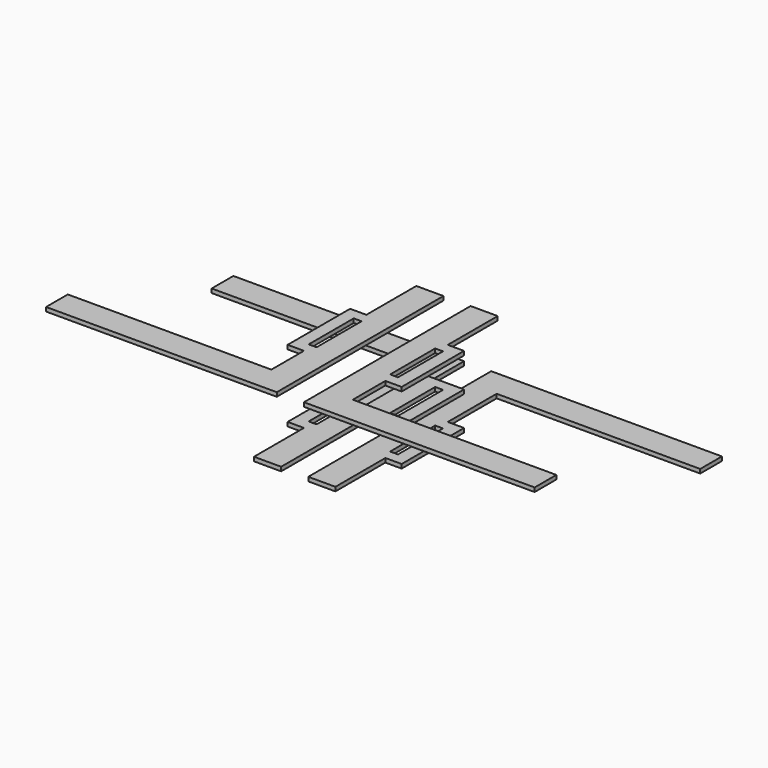
from build123d import *

# Parameters (mm, degrees)
F0_W      = 32
F0_H      = 57.5
F0_W_2    = 5.8
F0_H_2    = 41.5
F1_DEPTH  = 3
F3_W      = 5.8
F3_H      = 41.5
F3_W_2    = 20
F3_H_2    = 30
F3_H_3    = 46
F4_DEPTH  = 3
F9_W      = 20
F9_H      = 45
F9_W_2    = 5.8
F9_H_2    = 41.5
F9_H_3    = 46
F10_DEPTH = 3


# Not quite as in the source:
# - a feature names something its author has since deleted; it is built from what else it names


with BuildPart() as f1:
    # F0 (on Top) → F1 (new body)
    with BuildSketch(Plane.XY):
        with Locations((-4, 0)):
            Rectangle(F0_W, F0_H)
        Rectangle(F0_W_2, F0_H_2, mode=Mode.SUBTRACT)
    extrude(amount=F1_DEPTH)


with BuildPart() as f4:
    # F3 (on offset) → F4 (new body)
    with BuildSketch(Plane.XY.offset(25)):
        Polygon((0, 28.75), (-20, 28.75), (-20, -28.75), (0, -28.75), (12, -28.75), (12, 28.75), align=None)
        Rectangle(F3_W, F3_H, mode=Mode.SUBTRACT)
        with Locations((-10, -43.75)):
            Rectangle(F3_W_2, F3_H_2)
        Polygon((0, -58.75), (-20, -58.75), (-20, -78.75), (150, -78.75), (150, -58.75), align=None)
        with Locations((-10, 51.75)):
            Rectangle(F3_W_2, F3_H_3)
    extrude(amount=F4_DEPTH)


with BuildPart() as f6_1:
    # F6: instance of F4
    add(f4.part.mirror(Plane.YZ.offset(-30)))


with BuildPart() as f10:
    # F9 (on offset) → F10 (new body)
    with BuildSketch(Plane.XY.offset(-25)):
        Polygon((-20, 93.75), (-20, 73.75), (0, 73.75), (150, 73.75), (150, 93.75), align=None)
        with Locations((-10, 51.25)):
            Rectangle(F9_W, F9_H)
        Polygon((-20, 28.75), (-20, -28.75), (0, -28.75), (12, -28.75), (12, 28.75), (0, 28.75), align=None)
        Rectangle(F9_W_2, F9_H_2, mode=Mode.SUBTRACT)
        with Locations((-10, -51.75)):
            Rectangle(F9_W, F9_H_3)
    extrude(amount=F10_DEPTH)


with BuildPart() as f11_1:
    # F11: instance of F10
    add(f10.part.mirror(Plane.YZ.offset(-30)))


solid = Compound([f1.part, f4.part, f6_1.part, f10.part, f11_1.part])
